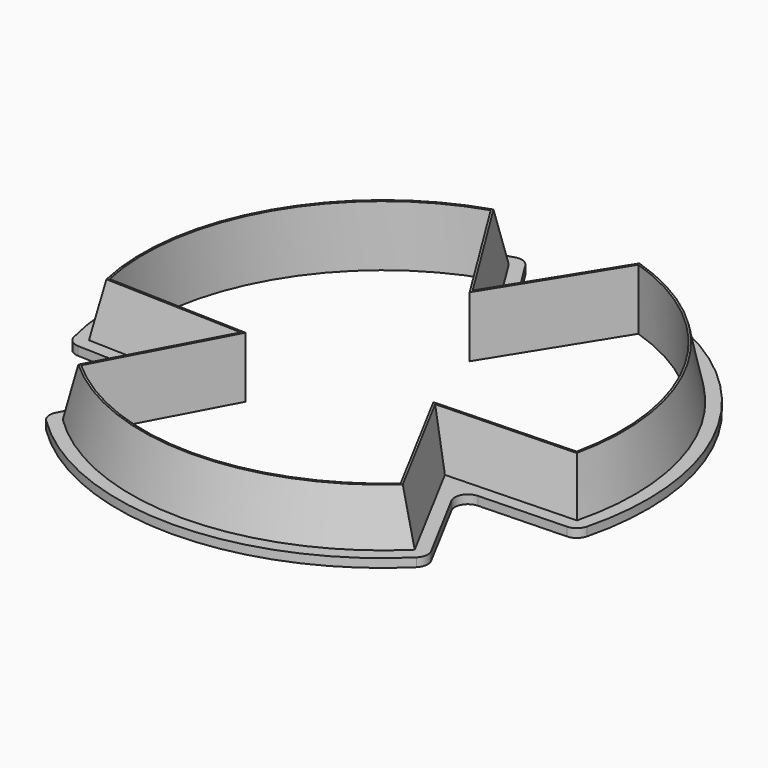
from build123d import *

# Parameters (mm, degrees)
F1_DEPTH = 12
F3_DEPTH = 2
F4_SIZE2 = 11.99999
F4_SIZE  = 2.550669
F5_R     = 3


# Not quite as in the source:
# - a fillet or chamfer is up to 0.001 mm smaller than in the source, because OpenCascade refuses the exact size


with BuildPart() as f1:
    # F0 (on Top) → F1 (new body)
    with BuildSketch(Plane.XY):
        with BuildLine():
            Line((15.6635716436, 55.8448970217), (0, 30.6775543541))
            Line((0, 30.6775543541), (-15.6635716436, 55.8448970217))
            ThreePointArc((-15.6635716436, 55.8448970217), (-50.2294734195, 29), (-56.1948853143, -14.3573975535))
            Line((-56.1948853143, -14.3573975535), (-26.5675413967, -15.3387771771))
            Line((-26.5675413967, -15.3387771771), (-40.5313136707, -41.4874994682))
            ThreePointArc((-40.5313136707, -41.4874994682), (0, -58), (40.5313136707, -41.4874994682))
            Line((40.5313136707, -41.4874994682), (26.5675413967, -15.3387771771))
            Line((26.5675413967, -15.3387771771), (56.1948853143, -14.3573975535))
            ThreePointArc((56.1948853143, -14.3573975535), (50.2294734195, 29), (15.6635716436, 55.8448970217))
        make_face()
        with BuildLine():
            ThreePointArc((-53.7981180404, -11.435142995), (-47.6313972081, 27.5), (-16.9959346906, 52.3081083962))
            Line((-16.9959346906, 52.3081083962), (0, 25))
            Line((0, 25), (16.9959346906, 52.3081083962))
            ThreePointArc((16.9959346906, 52.3081083962), (47.6313972081, 27.5), (53.7981180404, -11.435142995))
            Line((53.7981180404, -11.435142995), (21.6506350946, -12.5))
            Line((21.6506350946, -12.5), (36.8021833497, -40.8729654013))
            ThreePointArc((36.8021833497, -40.8729654013), (0, -55), (-36.8021833497, -40.8729654013))
            Line((-36.8021833497, -40.8729654013), (-21.6506350946, -12.5))
            Line((-21.6506350946, -12.5), (-53.7981180404, -11.435142995))
        make_face(mode=Mode.SUBTRACT)
    extrude(amount=F1_DEPTH)

    # F2 (on face) → F3 (join)
    with BuildSketch(Plane(origin=(0, 0, 0), x_dir=(1, 0, 0), z_dir=(0, 0, -1))):
        with BuildLine():
            Line((31.4844476987, 18.1775543541), (44.2174856505, 42.0215892459))
            ThreePointArc((44.2174856505, 42.0215892459), (0, 61), (-44.2174856505, 42.0215892459))
            Line((-44.2174856505, 42.0215892459), (-31.4844476987, 18.1775543541))
            Line((-31.4844476987, 18.1775543541), (-58.5005066196, 17.2826712419))
            ThreePointArc((-58.5005066196, 17.2826712419), (-52.8275496309, -30.5), (-14.2830209691, -59.3042604877))
            Line((-14.2830209691, -59.3042604877), (0, -36.3551087083))
            Line((0, -36.3551087083), (14.2830209691, -59.3042604877))
            ThreePointArc((14.2830209691, -59.3042604877), (52.8275496309, -30.5), (58.5005066196, 17.2826712419))
            Line((58.5005066196, 17.2826712419), (31.4844476987, 18.1775543541))
        make_face()
        with BuildLine():
            Line((-21.6506350946, 12.5), (-36.8021833497, 40.8729654013))
            ThreePointArc((-36.8021833497, 40.8729654013), (0, 55), (36.8021833497, 40.8729654013))
            Line((36.8021833497, 40.8729654013), (21.6506350946, 12.5))
            Line((21.6506350946, 12.5), (53.7981180404, 11.435142995))
            ThreePointArc((53.7981180404, 11.435142995), (47.6313972081, -27.5), (16.9959346906, -52.3081083962))
            Line((16.9959346906, -52.3081083962), (0, -25))
            Line((0, -25), (-16.9959346906, -52.3081083962))
            ThreePointArc((-16.9959346906, -52.3081083962), (-47.6313972081, -27.5), (-53.7981180404, 11.435142995))
            Line((-53.7981180404, 11.435142995), (-21.6506350946, 12.5))
        make_face(mode=Mode.SUBTRACT)
    extrude(amount=F3_DEPTH)

    # F4 (size 2.55067874 and 12 in the source; OpenCascade refuses exactly that, so slightly less here)
    f4_edges = [f1.edges().sort_by_distance(p)[0] for p in [
        (-41.381213, -14.848087, 12),
        (-33.549428, -28.413138, 12),
        (0, -58, 12),
        (-50.229473, 29, 12),
        (-7.831786, 43.261226, 12),
        (7.831786, 43.261226, 12),
        (50.229473, 29, 12),
        (41.381213, -14.848087, 12),
        (33.549428, -28.413138, 12),
    ]]
    f4_side = f1.faces().sort_by_distance((0, -56.37468, 12))[0]
    chamfer(f4_edges, length=F4_SIZE, length2=F4_SIZE2, reference=f4_side)

    # F5
    f5_edges = [f1.edges().sort_by_distance(p)[0] for p in [
        (-58.500507, -17.282671, -1),
        (-31.484448, -18.177554, -1),
        (-44.217486, -42.021589, -1),
        (44.217486, -42.021589, -1),
        (31.484448, -18.177554, -1),
        (58.500507, -17.282671, -1),
        (14.283021, 59.30426, -1),
        (0, 36.355109, -1),
        (-14.283021, 59.30426, -1),
    ]]
    fillet(f5_edges, radius=F5_R)


solid = f1.part
